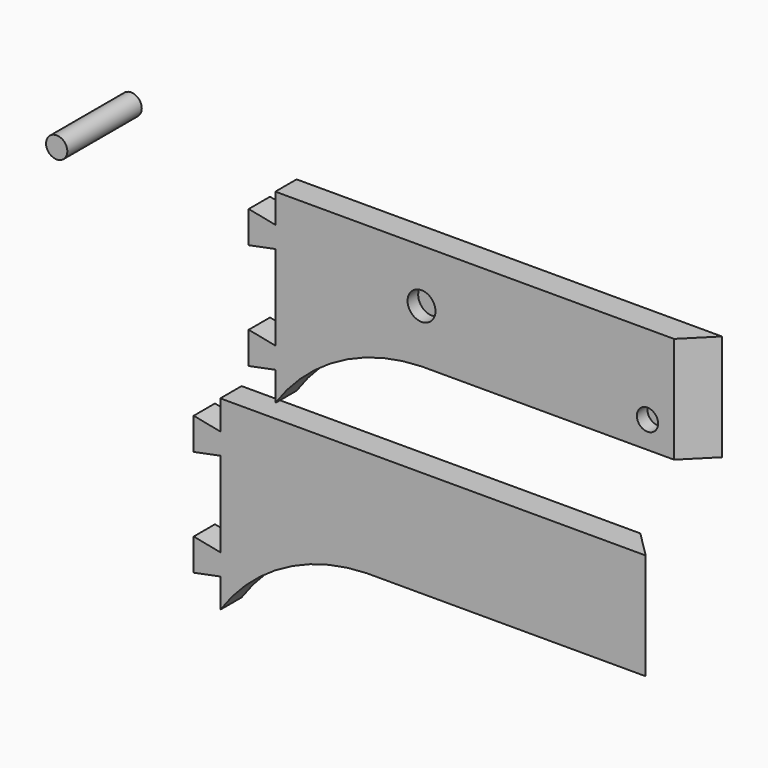
from build123d import *

# Parameters (mm, degrees)
F1_DEPTH  = 10
F2_R      = 5.25
F2_R_2    = 4
F3_DEPTH  = 5
F4_SIZE   = 9.99999
F6_DEPTH  = 10
F8_START  = -5
F7_R      = 5.25
F7_R_2    = 4
F8_DEPTH  = 5
F9_SIZE   = 9.99999
F10_R     = 4
F11_DEPTH = 35


# Not quite as in the source:
# - a fillet or chamfer is up to 0.001 mm smaller than in the source, because OpenCascade refuses the exact size


with BuildPart() as f1:
    # F0 (on Front) → F1 (new body)
    with BuildSketch(Plane.XZ):
        with BuildLine():
            ThreePointArc((10, -30), (33.8771457744, -8.3581005863), (65, 0))
            Line((65, 0), (170, 0))
            Line((170, 0), (170, 40))
            Line((170, 40), (10, 40))
            Line((10, 40), (10, 29))
            Line((10, 29), (0, 31))
            Line((0, 31), (0, 19))
            Line((0, 19), (10, 21))
            Line((10, 21), (10, -11))
            Line((10, -11), (0, -9))
            Line((0, -9), (0, -21))
            Line((0, -21), (10, -19))
            Line((10, -19), (10, -30))
        make_face()
    extrude(amount=F1_DEPTH)

    # F2 (on face) → F3 (cut)
    with BuildSketch(Plane.XZ.offset(10)):
        with Locations((65, 20)):
            Circle(F2_R)
        with Locations((150, 10)):
            Circle(F2_R_2)
    extrude(amount=-F3_DEPTH, mode=Mode.SUBTRACT)

    # F4 (size 10 in the source; OpenCascade refuses exactly that, so slightly less here)
    f4_edges = [f1.edges().sort_by_distance(p)[0] for p in [
        (170, -10, 20),
    ]]
    chamfer(f4_edges, length=F4_SIZE)


with BuildPart() as f6:
    # F5 (on Front) → F6 (new body)
    with BuildSketch(Plane.XZ):
        with BuildLine():
            ThreePointArc((-10.6844227825, -105.189197356), (13.1927229919, -83.5472979423), (44.3155772175, -75.189197356))
            Line((44.3155772175, -75.189197356), (149.3155772175, -75.189197356))
            Line((149.3155772175, -75.189197356), (149.3155772175, -35.189197356))
            Line((149.3155772175, -35.189197356), (-10.6844227825, -35.189197356))
            Line((-10.6844227825, -35.189197356), (-10.6844227825, -46.189197356))
            Line((-10.6844227825, -46.189197356), (-20.6844227825, -44.189197356))
            Line((-20.6844227825, -44.189197356), (-20.6844227825, -56.189197356))
            Line((-20.6844227825, -56.189197356), (-10.6844227825, -54.189197356))
            Line((-10.6844227825, -54.189197356), (-10.6844227825, -86.189197356))
            Line((-10.6844227825, -86.189197356), (-20.6844227825, -84.189197356))
            Line((-20.6844227825, -84.189197356), (-20.6844227825, -96.189197356))
            Line((-20.6844227825, -96.189197356), (-10.6844227825, -94.189197356))
            Line((-10.6844227825, -94.189197356), (-10.6844227825, -105.189197356))
        make_face()
    extrude(amount=F6_DEPTH)

    # F7 (on face) → F8 (cut)
    with BuildSketch(Plane.XZ.offset(10).offset(F8_START)):
        with Locations((44.3155772175, -55.189197356)):
            Circle(F7_R)
        with Locations((129.3155772175, -65.189197356)):
            Circle(F7_R_2)
    extrude(amount=-F8_DEPTH, mode=Mode.SUBTRACT)

    # F9 (size 10 in the source; OpenCascade refuses exactly that, so slightly less here)
    f9_edges = [f6.edges().sort_by_distance(p)[0] for p in [
        (149.315577, 0, -55.189197),
    ]]
    chamfer(f9_edges, length=F9_SIZE)


with BuildPart() as f11:
    # F10 (on Front) → F11 (new body)
    with BuildSketch(Plane.XZ):
        with Locations((-52.2351078689, 44.5644445717)):
            Circle(F10_R)
    extrude(amount=F11_DEPTH)


solid = Compound([f1.part, f6.part, f11.part])
